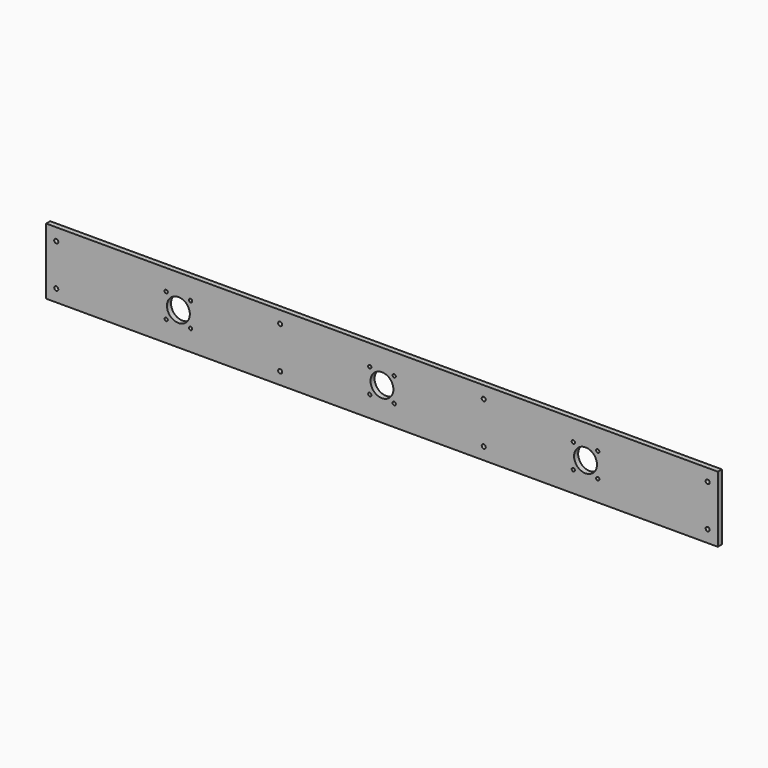
from build123d import *

# Parameters (mm, degrees)
F0_W     = 838.2
F0_H     = 82.55
F1_DEPTH = 6.35
F3_DEPTH = 6.35
F5_DEPTH = 6.35


# Not quite as in the source:
# - a pattern or mirror of a feature is missing from the dataset's text; its kind, count and spacing are read off the source's solid


with BuildPart() as f1:
    # F0 (on Front) → F1 (new body)
    with BuildSketch(Plane.XZ):
        Rectangle(F0_W, F0_H)
    extrude(amount=F1_DEPTH)

    # F2 (on face) → F3 (cut, through all)
    with BuildSketch(Plane.XZ.offset(6.35)):
        with BuildLine():
            ThreePointArc((-267.208, 15.24), (-270.6768409794, 16.6768409794), (-269.24, 13.208))
            Line((-269.24, 13.208), (-269.24, 15.24))
            Line((-269.24, 15.24), (-267.208, 15.24))
        make_face()
        with BuildLine():
            Line((-269.24, 15.24), (-269.24, 13.208))
            ThreePointArc((-269.24, 13.208), (-267.8031590206, 13.8031590206), (-267.208, 15.24))
            Line((-267.208, 15.24), (-269.24, 15.24))
        make_face()
        with BuildLine():
            Line((-254, 0), (-268.2875, 0))
            ThreePointArc((-268.2875, 0), (-254, -14.2875), (-239.7125, 0))
            ThreePointArc((-239.7125, 0), (-243.8972118638, 10.1027881362), (-254, 14.2875))
            Line((-254, 14.2875), (-254, 0))
        make_face()
        with BuildLine():
            ThreePointArc((-254, 14.2875), (-264.1027881362, 10.1027881362), (-268.2875, 0))
            Line((-268.2875, 0), (-254, 0))
            Line((-254, 0), (-254, 14.2875))
        make_face()
        with BuildLine():
            Line((-269.24, -15.24), (-269.24, -13.208))
            ThreePointArc((-269.24, -13.208), (-270.6768409794, -16.6768409794), (-267.208, -15.24))
            Line((-267.208, -15.24), (-269.24, -15.24))
        make_face()
        with BuildLine():
            ThreePointArc((-267.208, -15.24), (-267.8031590206, -13.8031590206), (-269.24, -13.208))
            Line((-269.24, -13.208), (-269.24, -15.24))
            Line((-269.24, -15.24), (-267.208, -15.24))
        make_face()
        with BuildLine():
            Line((-238.76, -15.24), (-240.792, -15.24))
            ThreePointArc((-240.792, -15.24), (-238.76, -17.272), (-236.728, -15.24))
            ThreePointArc((-236.728, -15.24), (-237.3231590206, -13.8031590206), (-238.76, -13.208))
            Line((-238.76, -13.208), (-238.76, -15.24))
        make_face()
        with BuildLine():
            ThreePointArc((-238.76, -13.208), (-240.1968409794, -13.8031590206), (-240.792, -15.24))
            Line((-240.792, -15.24), (-238.76, -15.24))
            Line((-238.76, -15.24), (-238.76, -13.208))
        make_face()
        with BuildLine():
            ThreePointArc((-236.728, 15.24), (-240.1968409794, 16.6768409794), (-238.76, 13.208))
            ThreePointArc((-238.76, 13.208), (-237.3231590206, 13.8031590206), (-236.728, 15.24))
        make_face()
        with BuildLine():
            ThreePointArc((14.2875, 0), (10.1027881362, 10.1027881362), (0, 14.2875))
            ThreePointArc((0, 14.2875), (-10.1027881362, -10.1027881362), (14.2875, 0))
        make_face()
        with BuildLine():
            Line((15.24, -15.24), (13.208, -15.24))
            ThreePointArc((13.208, -15.24), (15.24, -17.272), (17.272, -15.24))
            ThreePointArc((17.272, -15.24), (16.6768409794, -13.8031590206), (15.24, -13.208))
            Line((15.24, -13.208), (15.24, -15.24))
        make_face()
        with BuildLine():
            ThreePointArc((15.24, -13.208), (13.8031590206, -13.8031590206), (13.208, -15.24))
            Line((13.208, -15.24), (15.24, -15.24))
            Line((15.24, -15.24), (15.24, -13.208))
        make_face()
        with BuildLine():
            ThreePointArc((17.272, 15.24), (13.8031590206, 16.6768409794), (15.24, 13.208))
            ThreePointArc((15.24, 13.208), (16.6768409794, 13.8031590206), (17.272, 15.24))
        make_face()
        with BuildLine():
            Line((-15.24, 15.24), (-13.208, 15.24))
            ThreePointArc((-13.208, 15.24), (-16.6768409794, 16.6768409794), (-15.24, 13.208))
            Line((-15.24, 13.208), (-15.24, 15.24))
        make_face()
        with BuildLine():
            ThreePointArc((-15.24, 13.208), (-13.8031590206, 13.8031590206), (-13.208, 15.24))
            Line((-13.208, 15.24), (-15.24, 15.24))
            Line((-15.24, 15.24), (-15.24, 13.208))
        make_face()
        with BuildLine():
            Line((-15.24, -15.24), (-15.24, -13.208))
            ThreePointArc((-15.24, -13.208), (-16.6768409794, -16.6768409794), (-13.208, -15.24))
            Line((-13.208, -15.24), (-15.24, -15.24))
        make_face()
        with BuildLine():
            ThreePointArc((-13.208, -15.24), (-13.8031590206, -13.8031590206), (-15.24, -13.208))
            Line((-15.24, -13.208), (-15.24, -15.24))
            Line((-15.24, -15.24), (-13.208, -15.24))
        make_face()
    f3 = extrude(amount=-F3_DEPTH, mode=Mode.SUBTRACT)

    # F3_copies: F3 across plane
    add(f3.mirror(Plane(origin=(0, 0, 0), x_dir=(0, 0, 1), z_dir=(1, 0, 0))), mode=Mode.SUBTRACT)

    # F4 (on face) → F5 (cut, through all)
    with BuildSketch(Plane.XZ.offset(6.35)):
        with BuildLine():
            ThreePointArc((-403.86, 26.035), (-404.6039487758, 27.8310512242), (-406.4, 28.575))
            Line((-406.4, 28.575), (-406.4, 23.495))
            ThreePointArc((-406.4, 23.495), (-404.6039487758, 24.2389487758), (-403.86, 26.035))
        make_face()
        with BuildLine():
            ThreePointArc((-403.86, -26.035), (-404.6039487758, -24.2389487758), (-406.4, -23.495))
            Line((-406.4, -23.495), (-406.4, -28.575))
            ThreePointArc((-406.4, -28.575), (-404.6039487758, -27.8310512242), (-403.86, -26.035))
        make_face()
        with BuildLine():
            Line((-406.4, -28.575), (-406.4, -23.495))
            ThreePointArc((-406.4, -23.495), (-408.94, -26.035), (-406.4, -28.575))
        make_face()
        with BuildLine():
            Line((-406.4, 23.495), (-406.4, 28.575))
            ThreePointArc((-406.4, 28.575), (-408.94, 26.035), (-406.4, 23.495))
        make_face()
        with BuildLine():
            ThreePointArc((-124.46, 26.035), (-125.2039487758, 27.8310512242), (-127, 28.575))
            Line((-127, 28.575), (-127, 23.495))
            ThreePointArc((-127, 23.495), (-125.2039487758, 24.2389487758), (-124.46, 26.035))
        make_face()
        with BuildLine():
            ThreePointArc((-124.46, -26.035), (-125.2039487758, -24.2389487758), (-127, -23.495))
            Line((-127, -23.495), (-127, -28.575))
            ThreePointArc((-127, -28.575), (-125.2039487758, -27.8310512242), (-124.46, -26.035))
        make_face()
        with BuildLine():
            Line((-127, -28.575), (-127, -23.495))
            ThreePointArc((-127, -23.495), (-129.54, -26.035), (-127, -28.575))
        make_face()
        with BuildLine():
            Line((-127, 23.495), (-127, 28.575))
            ThreePointArc((-127, 28.575), (-129.54, 26.035), (-127, 23.495))
        make_face()
    f5 = extrude(amount=-F5_DEPTH, mode=Mode.SUBTRACT)

    # F5_copies: F5 across plane
    add(f5.mirror(Plane(origin=(0, 0, 0), x_dir=(0, 0, 1), z_dir=(1, 0, 0))), mode=Mode.SUBTRACT)


solid = f1.part
